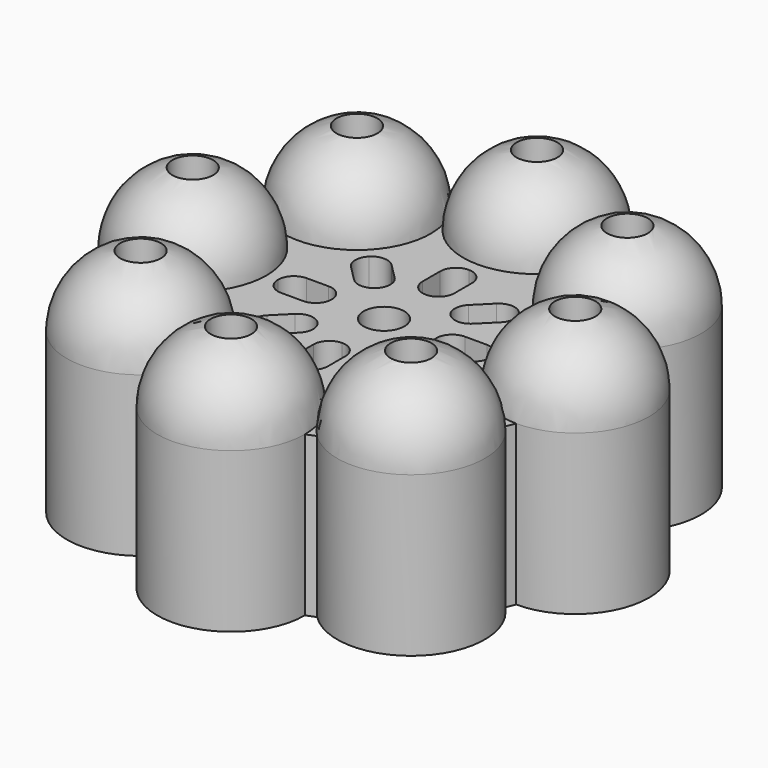
from build123d import *

# Parameters (mm, degrees)
F0_R            = 8.375
F0_R_2          = 3.2
F1_DEPTH        = 25
F3_ANGLE        = 180
F3_COPIES_COUNT = 8
F4_R            = 3.2
F5_DEPTH        = 36.576
F5_COPIES_COUNT = 8


# Not quite as in the source:
# - a pattern or mirror of a feature is missing from the dataset's text; its kind, count and spacing are read off the source's solid


with BuildPart() as f1:
    # F0 (on Top) → F1 (new body)
    with BuildSketch(Plane.XY):
        with BuildLine():
            Line((13.0284424434, 29.3979644278), (11.575, 30))
            ThreePointArc((11.575, 30), (0, 41.575), (-11.575, 30))
            Line((-11.575, 30), (-13.0284424434, 29.3979644278))
            ThreePointArc((-13.0284424434, 29.3979644278), (-29.3979644278, 29.3979644278), (-29.3979644278, 13.0284424434))
            Line((-29.3979644278, 13.0284424434), (-30, 11.575))
            ThreePointArc((-30, 11.575), (-41.575, 0), (-30, -11.575))
            Line((-30, -11.575), (-29.3979644278, -13.0284424434))
            ThreePointArc((-29.3979644278, -13.0284424434), (-29.3979644278, -29.3979644278), (-13.0284424434, -29.3979644278))
            Line((-13.0284424434, -29.3979644278), (-11.575, -30))
            ThreePointArc((-11.575, -30), (0, -41.575), (11.575, -30))
            Line((11.575, -30), (13.0284424434, -29.3979644278))
            ThreePointArc((13.0284424434, -29.3979644278), (29.3979644278, -29.3979644278), (29.3979644278, -13.0284424434))
            Line((29.3979644278, -13.0284424434), (30, -11.575))
            ThreePointArc((30, -11.575), (41.575, 0), (30, 11.575))
            Line((30, 11.575), (29.3979644278, 13.0284424434))
            ThreePointArc((29.3979644278, 13.0284424434), (29.3979644278, 29.3979644278), (13.0284424434, 29.3979644278))
        make_face()
        with Locations((-21.2132034356, -21.2132034356)):
            Circle(F0_R, mode=Mode.SUBTRACT)
        with BuildLine():
            ThreePointArc((-5.7982756057, -5.7982756057), (-5.0660425587, -7.5660425587), (-5.7982756057, -9.3338095117))
            Line((-5.7982756057, -9.3338095117), (-8.2201163313, -11.7556502372))
            ThreePointArc((-8.2201163313, -11.7556502372), (-9.9878832843, -12.4878832843), (-11.7556502372, -11.7556502372))
            ThreePointArc((-11.7556502372, -11.7556502372), (-12.4878832843, -9.9878832843), (-11.7556502372, -8.2201163313))
            Line((-11.7556502372, -8.2201163313), (-9.3338095117, -5.7982756057))
            ThreePointArc((-9.3338095117, -5.7982756057), (-7.5660425587, -5.0660425587), (-5.7982756057, -5.7982756057))
        make_face(mode=Mode.SUBTRACT)
        with Locations((0, -30)):
            Circle(F0_R, mode=Mode.SUBTRACT)
        with Locations((21.2132034356, -21.2132034356)):
            Circle(F0_R, mode=Mode.SUBTRACT)
        with BuildLine():
            ThreePointArc((0, -8.2), (1.767766953, -8.932233047), (2.5, -10.7))
            Line((2.5, -10.7), (2.5, -14.125))
            ThreePointArc((2.5, -14.125), (1.767766953, -15.892766953), (0, -16.625))
            ThreePointArc((0, -16.625), (-1.767766953, -15.892766953), (-2.5, -14.125))
            Line((-2.5, -14.125), (-2.5, -10.7))
            ThreePointArc((-2.5, -10.7), (-1.767766953, -8.932233047), (0, -8.2))
        make_face(mode=Mode.SUBTRACT)
        with BuildLine():
            ThreePointArc((5.7982756057, -5.7982756057), (7.5660425587, -5.0660425587), (9.3338095117, -5.7982756057))
            Line((9.3338095117, -5.7982756057), (11.7556502372, -8.2201163313))
            ThreePointArc((11.7556502372, -8.2201163313), (12.4878832843, -9.9878832843), (11.7556502372, -11.7556502372))
            ThreePointArc((11.7556502372, -11.7556502372), (9.9878832843, -12.4878832843), (8.2201163313, -11.7556502372))
            Line((8.2201163313, -11.7556502372), (5.7982756057, -9.3338095117))
            ThreePointArc((5.7982756057, -9.3338095117), (5.0660425587, -7.5660425587), (5.7982756057, -5.7982756057))
        make_face(mode=Mode.SUBTRACT)
        with Locations((-30, 0)):
            Circle(F0_R, mode=Mode.SUBTRACT)
        with BuildLine():
            ThreePointArc((-8.2, 0), (-8.932233047, -1.767766953), (-10.7, -2.5))
            Line((-10.7, -2.5), (-14.125, -2.5))
            ThreePointArc((-14.125, -2.5), (-15.892766953, -1.767766953), (-16.625, 0))
            ThreePointArc((-16.625, 0), (-15.892766953, 1.767766953), (-14.125, 2.5))
            Line((-14.125, 2.5), (-10.7, 2.5))
            ThreePointArc((-10.7, 2.5), (-8.932233047, 1.767766953), (-8.2, 0))
        make_face(mode=Mode.SUBTRACT)
        with BuildLine():
            ThreePointArc((-5.7982756057, 5.7982756057), (-7.5660425587, 5.0660425587), (-9.3338095117, 5.7982756057))
            Line((-9.3338095117, 5.7982756057), (-11.7556502372, 8.2201163313))
            ThreePointArc((-11.7556502372, 8.2201163313), (-12.4878832843, 9.9878832843), (-11.7556502372, 11.7556502372))
            ThreePointArc((-11.7556502372, 11.7556502372), (-9.9878832843, 12.4878832843), (-8.2201163313, 11.7556502372))
            Line((-8.2201163313, 11.7556502372), (-5.7982756057, 9.3338095117))
            ThreePointArc((-5.7982756057, 9.3338095117), (-5.0660425587, 7.5660425587), (-5.7982756057, 5.7982756057))
        make_face(mode=Mode.SUBTRACT)
        with Locations((-21.2132034356, 21.2132034356)):
            Circle(F0_R, mode=Mode.SUBTRACT)
        Circle(F0_R_2, mode=Mode.SUBTRACT)
        with BuildLine():
            ThreePointArc((5.7982756057, 5.7982756057), (5.0660425587, 7.5660425587), (5.7982756057, 9.3338095117))
            Line((5.7982756057, 9.3338095117), (8.2201163313, 11.7556502372))
            ThreePointArc((8.2201163313, 11.7556502372), (9.9878832843, 12.4878832843), (11.7556502372, 11.7556502372))
            ThreePointArc((11.7556502372, 11.7556502372), (12.4878832843, 9.9878832843), (11.7556502372, 8.2201163313))
            Line((11.7556502372, 8.2201163313), (9.3338095117, 5.7982756057))
            ThreePointArc((9.3338095117, 5.7982756057), (7.5660425587, 5.0660425587), (5.7982756057, 5.7982756057))
        make_face(mode=Mode.SUBTRACT)
        with BuildLine():
            ThreePointArc((8.2, 0), (8.932233047, 1.767766953), (10.7, 2.5))
            Line((10.7, 2.5), (14.125, 2.5))
            ThreePointArc((14.125, 2.5), (15.892766953, 1.767766953), (16.625, 0))
            ThreePointArc((16.625, 0), (15.892766953, -1.767766953), (14.125, -2.5))
            Line((14.125, -2.5), (10.7, -2.5))
            ThreePointArc((10.7, -2.5), (8.932233047, -1.767766953), (8.2, 0))
        make_face(mode=Mode.SUBTRACT)
        with BuildLine():
            Line((2.5, 14.125), (2.5, 10.7))
            ThreePointArc((2.5, 10.7), (1.767766953, 8.932233047), (0, 8.2))
            ThreePointArc((0, 8.2), (-1.767766953, 8.932233047), (-2.5, 10.7))
            Line((-2.5, 10.7), (-2.5, 14.125))
            ThreePointArc((-2.5, 14.125), (-1.767766953, 15.892766953), (0, 16.625))
            ThreePointArc((0, 16.625), (1.767766953, 15.892766953), (2.5, 14.125))
        make_face(mode=Mode.SUBTRACT)
        with Locations((30, 0)):
            Circle(F0_R, mode=Mode.SUBTRACT)
        with Locations((0, 30)):
            Circle(F0_R, mode=Mode.SUBTRACT)
        with Locations((21.2132034356, 21.2132034356)):
            Circle(F0_R, mode=Mode.SUBTRACT)
    extrude(amount=F1_DEPTH)

    # F2 (on face) → F3 (revolve)
    with BuildSketch(Plane.XY.offset(25)):
        with BuildLine():
            ThreePointArc((0, 18.425), (11.575, 30), (0, 41.575))
            Line((0, 41.575), (0, 38.375))
            ThreePointArc((0, 38.375), (8.375, 30), (0, 21.625))
            Line((0, 21.625), (0, 18.425))
        make_face()
    f3 = revolve(axis=Axis((0, 39.975, 25), (0, -1, 0)), revolution_arc=F3_ANGLE)

    # F3_copies: F3 ×8 about axis
    f3_copies_axis = Axis((0, 0, 0), (0, 0, 1))
    for i in range(1, F3_COPIES_COUNT):
        add(f3.rotate(f3_copies_axis, i * 360 / F3_COPIES_COUNT))

    # F4 (on Top) → F5 (cut, through all)
    with BuildSketch(Plane.XY):
        with Locations((0, 30)):
            Circle(F4_R)
    f5 = extrude(amount=F5_DEPTH, mode=Mode.SUBTRACT)

    # F5_copies: F5 ×8 about axis
    f5_copies_axis = Axis((0, 0, 0), (0, 0, 1))
    for i in range(1, F5_COPIES_COUNT):
        add(f5.rotate(f5_copies_axis, i * 360 / F5_COPIES_COUNT), mode=Mode.SUBTRACT)


solid = f1.part
